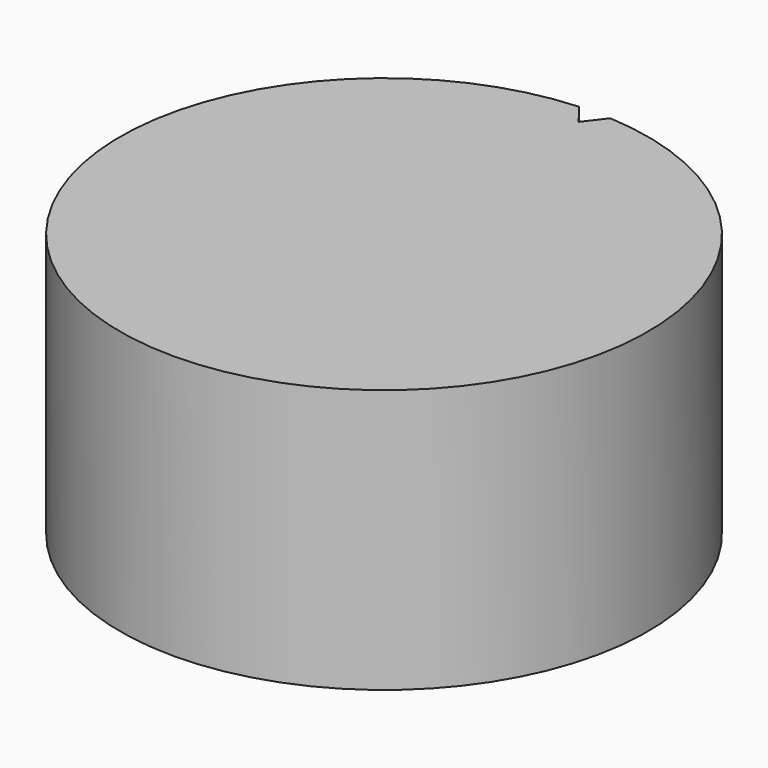
from build123d import *

# Parameters (mm, degrees)
F1_DEPTH = 25
F2_DEPTH = 30


with BuildPart() as f1:
    # F0 (on Top) → F1 (new body)
    with BuildSketch(Plane.XY):
        with BuildLine():
            ThreePointArc((-1.477426165, 24.9563060553), (-17.1473663557, -18.1925211849), (25, 0))
            ThreePointArc((25, 0), (18.1925211849, 17.1473663557), (1.477426165, 24.9563060553))
            Line((1.477426165, 24.9563060553), (0, 23.0396687984))
            Line((0, 23.0396687984), (-1.477426165, 24.9563060553))
        make_face()
    extrude(amount=F1_DEPTH)

    # F0 (on Top) → F2 (cut)
    with BuildSketch(Plane.XY):
        with BuildLine():
            ThreePointArc((0, 25), (-0.7390360671, 24.9890741263), (-1.477426165, 24.9563060553))
            Line((-1.477426165, 24.9563060553), (0, 23.0396687984))
            Line((0, 23.0396687984), (0, 25))
        make_face()
        with BuildLine():
            Line((0, 23.0396687984), (1.477426165, 24.9563060553))
            ThreePointArc((1.477426165, 24.9563060553), (0.7390360671, 24.9890741263), (0, 25))
            Line((0, 25), (0, 23.0396687984))
        make_face()
    extrude(amount=F2_DEPTH, mode=Mode.SUBTRACT)


solid = f1.part
